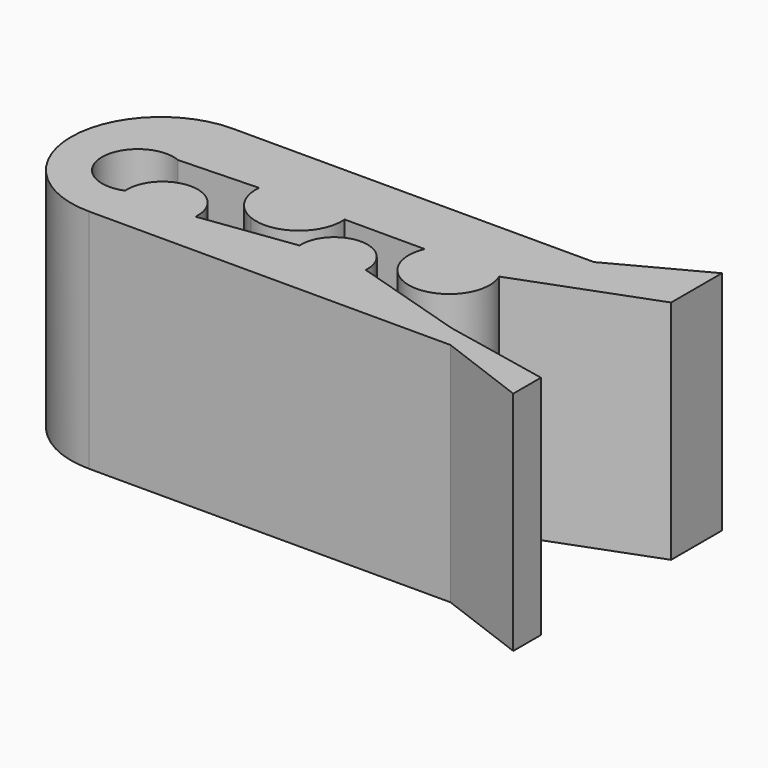
from build123d import *

# Parameters (mm, degrees)
F1_DEPTH = 25
F4_DEPTH = 25
F5_DEPTH = 25


with BuildPart() as f1:
    # F0 (on Top) → F1 (new body)
    with BuildSketch(Plane.XY):
        with BuildLine():
            ThreePointArc((0, -25.2255909145), (-9.9045261741, -35.1301170886), (0, -45.0346432626))
            Line((0, -45.0346432626), (39.8768223822, -45.0346432626))
            Line((39.8768223822, -45.0346432626), (49.781344831, -48.7488396466))
            Line((49.781344831, -48.7488396466), (49.781344831, -19.9638102204))
            Line((49.781344831, -19.9638102204), (39.8768223822, -25.2255909145))
            Line((39.8768223822, -25.2255909145), (0, -25.2255909145))
        make_face()
    extrude(amount=F1_DEPTH)

    # F2 (on face) → F4 (join)
    with BuildSketch(Plane.XY.offset(25)):
        with BuildLine():
            Line((39.8768223822, -25.2255909145), (0, -25.2255909145))
            ThreePointArc((0, -25.2255909145), (-9.9045261741, -35.1301170886), (0, -45.0346432626))
            Line((0, -45.0346432626), (39.8768223822, -45.0346432626))
            Line((39.8768223822, -45.0346432626), (49.781344831, -48.7488396466))
            Line((49.781344831, -48.7488396466), (49.781344831, -19.9638102204))
            Line((49.781344831, -19.9638102204), (39.8768223822, -25.2255909145))
        make_face()
    extrude(amount=-F4_DEPTH)

    # F3 (on face) → F5 (cut)
    with BuildSketch(Plane.XY.offset(25)):
        with BuildLine():
            Line((8.6823031306, -32.4443913996), (0, -32.7490344644))
            ThreePointArc((0, -32.7490344644), (-5.4739792074, -36.4047400653), (0, -40.0604456663))
            ThreePointArc((0, -40.0604456663), (2.12452123, -36.2934819265), (6.4182874872, -36.8103741808))
            ThreePointArc((6.4182874872, -36.8103741808), (7.8913776241, -38.1191729594), (8.6357264586, -39.9436985434))
            Line((8.6357264586, -39.9436985434), (18.1262083352, -38.6662621896))
            ThreePointArc((18.1262083352, -38.6662621896), (21.7819157988, -34.7755161234), (25.4376232624, -38.6662621896))
            Line((25.4376232624, -38.6662621896), (37.927955389, -42.4975827336))
            Line((37.927955389, -42.4975827336), (49.781344831, -44.9290481875))
            Line((49.781344831, -44.9290481875), (49.781344831, -26.9712014124))
            Line((49.781344831, -26.9712014124), (35.1861715317, -32.4443913996))
            ThreePointArc((35.1861715317, -32.4443913996), (31.0735022649, -38.6662621896), (26.9608329982, -32.4443913996))
            Line((26.9608329982, -32.4443913996), (19.0401375294, -32.4443913996))
            ThreePointArc((19.0401375294, -32.4443913996), (16.6761777926, -36.8994118679), (11.6438215498, -37.2324338722))
            ThreePointArc((11.6438215498, -37.2324338722), (9.374780297, -35.3259838728), (8.6823031306, -32.4443913996))
        make_face()
        with BuildLine():
            ThreePointArc((8.6357264586, -39.9436985434), (7.8913776241, -38.1191729594), (6.4182874872, -36.8103741808))
            ThreePointArc((6.4182874872, -36.8103741808), (7.4813175027, -38.2742394866), (7.7683748677, -40.0604456663))
            Line((7.7683748677, -40.0604456663), (8.6357264586, -39.9436985434))
        make_face()
        with BuildLine():
            ThreePointArc((18.1262083352, -32.4443913996), (16.2192131955, -36.6447435476), (11.6438215498, -37.2324338722))
            ThreePointArc((11.6438215498, -37.2324338722), (16.6761777926, -36.8994118679), (19.0401375294, -32.4443913996))
            Line((19.0401375294, -32.4443913996), (18.1262083352, -32.4443913996))
        make_face()
    extrude(amount=-F5_DEPTH, mode=Mode.SUBTRACT)


solid = f1.part
